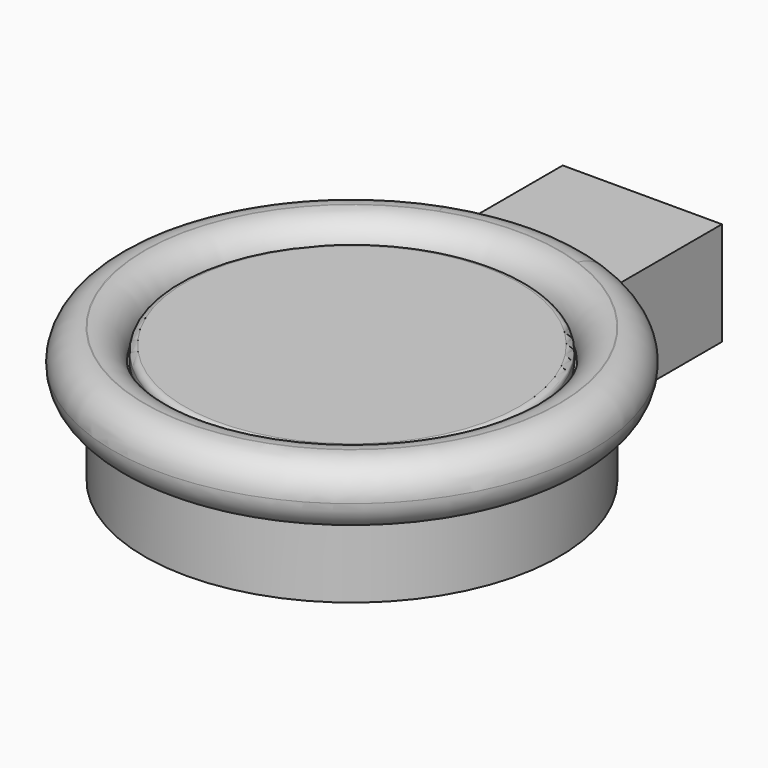
from build123d import *

# Parameters (mm, degrees)
F0_R     = 7.5
F0_R_2   = 83.55
F0_R_3   = 82.55
F3_DEPTH = 34.4
F4_DEPTH = 14.8
F5_START = 14.8
F5_DEPTH = 14.8
F6_R     = 14.79
F7_START = 14.8
F7_DEPTH = 7.4
F8_R     = 3


# Not quite as in the source:
# - a feature names something its author has since deleted; it is built from what else it names


with BuildPart() as f3:
    # F0 (on Top) → F3 (new body)
    with BuildSketch(Plane.XY):
        with BuildLine():
            ThreePointArc((-37.8333333333, 107.0088262196), (0, 113.5), (37.8333333333, 107.0088262196))
            Line((37.8333333333, 107.0088262196), (37.8333333333, 172.5))
            Line((37.8333333333, 172.5), (-37.8333333333, 172.5))
            Line((-37.8333333333, 172.5), (-37.8333333333, 107.0088262196))
        make_face()
        with Locations((0, 157.5)):
            Circle(F0_R, mode=Mode.SUBTRACT)
        with BuildLine():
            Line((37.8333333333, 90.9715038564), (37.8333333333, 107.0088262196))
            ThreePointArc((37.8333333333, 107.0088262196), (0, 113.5), (-37.8333333333, 107.0088262196))
            Line((-37.8333333333, 107.0088262196), (-37.8333333333, 90.9715038564))
            ThreePointArc((-37.8333333333, 90.9715038564), (0, 98.525), (37.8333333333, 90.9715038564))
        make_face()
        with BuildLine():
            ThreePointArc((98.525, 0), (81.9594558049, 54.6792760483), (37.8333333333, 90.9715038564))
            ThreePointArc((37.8333333333, 90.9715038564), (0, 98.525), (-37.8333333333, 90.9715038564))
            ThreePointArc((-37.8333333333, 90.9715038564), (-54.6792760483, -81.9594558049), (98.525, 0))
        make_face()
        Circle(F0_R_2, mode=Mode.SUBTRACT)
        Circle(F0_R_2)
        Circle(F0_R_3, mode=Mode.SUBTRACT)
        Circle(F0_R_3)
    extrude(amount=-F3_DEPTH)

    # F0 (on Top) → F4 (join)
    with BuildSketch(Plane.XY):
        with BuildLine():
            ThreePointArc((-37.8333333333, 107.0088262196), (-65.529255553, -92.6723619353), (113.5, 0))
            ThreePointArc((113.5, 0), (92.6723619353, 65.529255553), (37.8333333333, 107.0088262196))
            Line((37.8333333333, 107.0088262196), (37.8333333333, 90.9715038564))
            ThreePointArc((37.8333333333, 90.9715038564), (81.9594558049, 54.6792760483), (98.525, 0))
            ThreePointArc((98.525, 0), (-54.6792760483, -81.9594558049), (-37.8333333333, 90.9715038564))
            Line((-37.8333333333, 90.9715038564), (-37.8333333333, 107.0088262196))
        make_face()
        with BuildLine():
            ThreePointArc((98.525, 0), (81.9594558049, 54.6792760483), (37.8333333333, 90.9715038564))
            ThreePointArc((37.8333333333, 90.9715038564), (0, 98.525), (-37.8333333333, 90.9715038564))
            ThreePointArc((-37.8333333333, 90.9715038564), (-54.6792760483, -81.9594558049), (98.525, 0))
        make_face()
        Circle(F0_R_2, mode=Mode.SUBTRACT)
        Circle(F0_R_2)
        Circle(F0_R_3, mode=Mode.SUBTRACT)
        Circle(F0_R_3)
        with BuildLine():
            Line((37.8333333333, 90.9715038564), (37.8333333333, 107.0088262196))
            ThreePointArc((37.8333333333, 107.0088262196), (0, 113.5), (-37.8333333333, 107.0088262196))
            Line((-37.8333333333, 107.0088262196), (-37.8333333333, 90.9715038564))
            ThreePointArc((-37.8333333333, 90.9715038564), (0, 98.525), (37.8333333333, 90.9715038564))
        make_face()
        with BuildLine():
            ThreePointArc((-37.8333333333, 107.0088262196), (0, 113.5), (37.8333333333, 107.0088262196))
            Line((37.8333333333, 107.0088262196), (37.8333333333, 172.5))
            Line((37.8333333333, 172.5), (-37.8333333333, 172.5))
            Line((-37.8333333333, 172.5), (-37.8333333333, 107.0088262196))
        make_face()
        with Locations((0, 157.5)):
            Circle(F0_R, mode=Mode.SUBTRACT)
        with Locations((0, 157.5)):
            Circle(F0_R)
    extrude(amount=F4_DEPTH)

    # F0 (on Top) → F5 (join)
    with BuildSketch(Plane.XY.offset(F5_START)):
        with BuildLine():
            ThreePointArc((-37.8333333333, 107.0088262196), (-65.529255553, -92.6723619353), (113.5, 0))
            ThreePointArc((113.5, 0), (92.6723619353, 65.529255553), (37.8333333333, 107.0088262196))
            Line((37.8333333333, 107.0088262196), (37.8333333333, 90.9715038564))
            ThreePointArc((37.8333333333, 90.9715038564), (81.9594558049, 54.6792760483), (98.525, 0))
            ThreePointArc((98.525, 0), (-54.6792760483, -81.9594558049), (-37.8333333333, 90.9715038564))
            Line((-37.8333333333, 90.9715038564), (-37.8333333333, 107.0088262196))
        make_face()
        with BuildLine():
            ThreePointArc((98.525, 0), (81.9594558049, 54.6792760483), (37.8333333333, 90.9715038564))
            ThreePointArc((37.8333333333, 90.9715038564), (0, 98.525), (-37.8333333333, 90.9715038564))
            ThreePointArc((-37.8333333333, 90.9715038564), (-54.6792760483, -81.9594558049), (98.525, 0))
        make_face()
        Circle(F0_R_2, mode=Mode.SUBTRACT)
        with BuildLine():
            Line((37.8333333333, 90.9715038564), (37.8333333333, 107.0088262196))
            ThreePointArc((37.8333333333, 107.0088262196), (0, 113.5), (-37.8333333333, 107.0088262196))
            Line((-37.8333333333, 107.0088262196), (-37.8333333333, 90.9715038564))
            ThreePointArc((-37.8333333333, 90.9715038564), (0, 98.525), (37.8333333333, 90.9715038564))
        make_face()
    extrude(amount=F5_DEPTH)

    # F6
    f6_edges = [f3.edges().sort_by_distance(p)[0] for p in [
        (-37.833333, -107.008826, 29.6),
        (-83.55, 0, 29.6),
        (0, -113.5, 0),
    ]]
    fillet(f6_edges, radius=F6_R)


with BuildPart() as f7:
    # F0 (on Top) → F7 (new body)
    with BuildSketch(Plane.XY.offset(F7_START)):
        Circle(F0_R_3)
    extrude(amount=F7_DEPTH)

    # F8
    f8_edges = [f7.edges().sort_by_distance(p)[0] for p in [
        (-82.55, 0, 22.2),
    ]]
    fillet(f8_edges, radius=F8_R)


solid = Compound([f3.part, f7.part])
